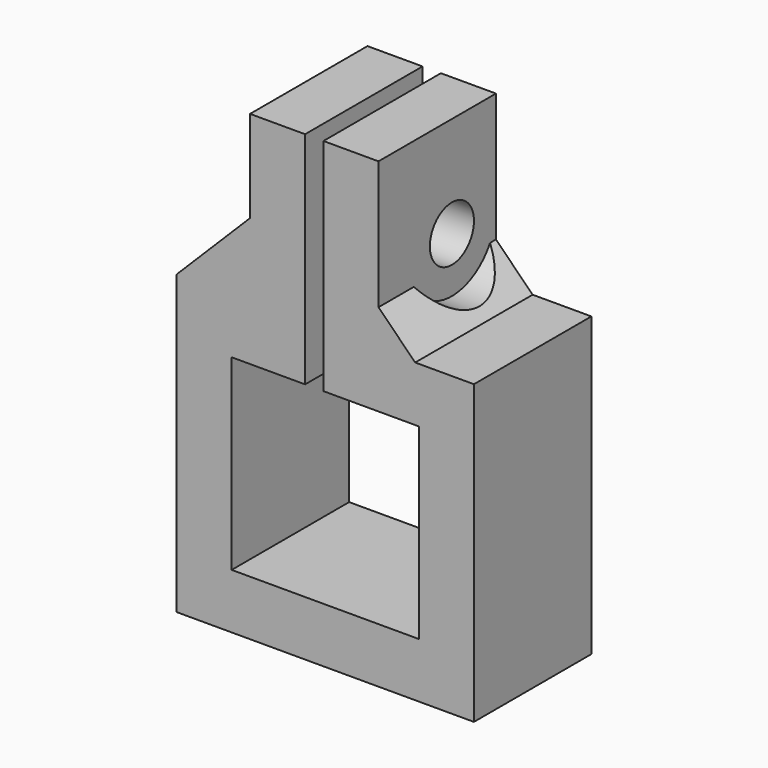
from build123d import *

# Parameters (mm, degrees)
F1_DEPTH = 8
F2_R     = 1.5
F3_DEPTH = 12.5
F4_SIZE  = 1.99999
F5_R     = 3
F6_DEPTH = 4
F8_DEPTH = 2


# Not quite as in the source:
# - a fillet or chamfer is up to 0.001 mm smaller than in the source, because OpenCascade refuses the exact size


with BuildPart() as f1:
    # F0 (on Front) → F1 (new body)
    with BuildSketch(Plane.XZ):
        Polygon((5.1, 5.1), (5.1, -5.1), (-5.1, -5.1), (-5.1, 5.1), (-4.1, 5.1), (-1.1, 5.1), (-1.1, 8.1), (-1.1, 17.1), (-4.1, 17.1), (-4.1, 8.1), (-5.1, 8.1), (-8.1, 8.1), (-8.1, -8.1), (8.1, -8.1), (8.1, 8.1), (2.9, 8.1), (2.9, 17.1), (-0.1, 17.1), (-0.1, 8.1), (-0.1, 5.1), align=None)
    extrude(amount=F1_DEPTH)

    # F2 (on face) → F3 (cut, symmetric)
    with BuildSketch(Plane.YZ.offset(-1.1)):
        with Locations((-3, 11.6)):
            Circle(F2_R)
    extrude(amount=F3_DEPTH, both=True, mode=Mode.SUBTRACT)

    # F4 (size 2 in the source; OpenCascade refuses exactly that, so slightly less here)
    f4_edges = [f1.edges().sort_by_distance(p)[0] for p in [
        (2.9, -4, 8.1),
    ]]
    chamfer(f4_edges, length=F4_SIZE)

    # F5 (on face) → F6 (cut)
    with BuildSketch(Plane.YZ.offset(2.9)):
        with Locations((-3, 11.6)):
            Circle(F5_R)
    extrude(amount=F6_DEPTH, mode=Mode.SUBTRACT)

    # F7 (on face) → F8 (join)
    with BuildSketch(Plane.XZ.offset(8)):
        Polygon((-4.1, 12.1), (-8.1, 8.1), (-4.1, 8.1), align=None)
    extrude(amount=-F8_DEPTH)


solid = f1.part
